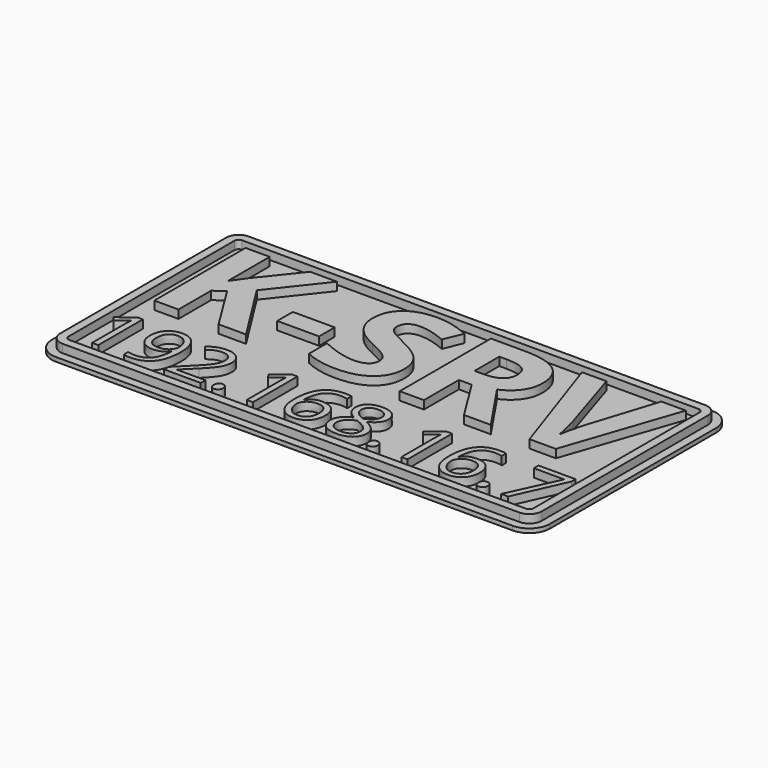
from build123d import *

# Parameters (mm, degrees)
F3_DEPTH       = 1
F4_TEXT_SIZE   = 38.4693822788
F4_TEXT_SIZE_2 = 18.798846053
F5_DEPTH       = 2


# Not quite as in the source:
# - a feature names something its author has since deleted; it is built from what else it names
# - Text() gives the source's letters only with a copy of the font that has no kerning and outlines rounded to 1/6400 em; it was checked with that copy


with BuildPart() as f3:
    # F2 (on Top) → F3 (new body)
    with BuildSketch(Plane.XY):
        with BuildLine():
            Line((55, 30), (-55, 30))
            ThreePointArc((-55, 30), (-58.5355339059, 28.5355339059), (-60, 25))
            Line((-60, 25), (-60, -25))
            ThreePointArc((-60, -25), (-58.5355339059, -28.5355339059), (-55, -30))
            Line((-55, -30), (55, -30))
            ThreePointArc((55, -30), (58.5355339059, -28.5355339059), (60, -25))
            Line((60, -25), (60, 25))
            ThreePointArc((60, 25), (58.5355339059, 28.5355339059), (55, 30))
        make_face()
    extrude(amount=F3_DEPTH)

    # F4 (on face) → F5 (join)
    with BuildSketch(Plane.XY.offset(1)):
        with BuildLine():
            Line((55, 28), (-55, 28))
            ThreePointArc((-55, 28), (-57.1213203436, 27.1213203436), (-58, 25))
            Line((-58, 25), (-58, -25))
            ThreePointArc((-58, -25), (-57.1213203436, -27.1213203436), (-55, -28))
            Line((-55, -28), (55, -28))
            ThreePointArc((55, -28), (57.1213203436, -27.1213203436), (58, -25))
            Line((58, -25), (58, 25))
            ThreePointArc((58, 25), (57.1213203436, 27.1213203436), (55, 28))
        make_face()
        with BuildLine():
            ThreePointArc((-56, 25), (-55.7071067812, 25.7071067812), (-55, 26))
            Line((-55, 26), (55, 26))
            ThreePointArc((55, 26), (55.7071067812, 25.7071067812), (56, 25))
            Line((56, 25), (56, -25))
            ThreePointArc((56, -25), (55.7071067812, -25.7071067812), (55, -26))
            Line((55, -26), (-55, -26))
            ThreePointArc((-55, -26), (-55.7071067812, -25.7071067812), (-56, -25))
            Line((-56, -25), (-56, 25))
        make_face(mode=Mode.SUBTRACT)
        with Locations((-56, -3.4770742636)):
            Text('K-SRV', F4_TEXT_SIZE, font='Open Sans', font_style=FontStyle.BOLD, text_align=(TextAlign.LEFT, TextAlign.BOTTOM))
        with Locations((-56, -24.2208809771)):
            Text('192.168.16.7', F4_TEXT_SIZE_2, font='Open Sans', text_align=(TextAlign.LEFT, TextAlign.BOTTOM))
    extrude(amount=F5_DEPTH)


solid = f3.part
